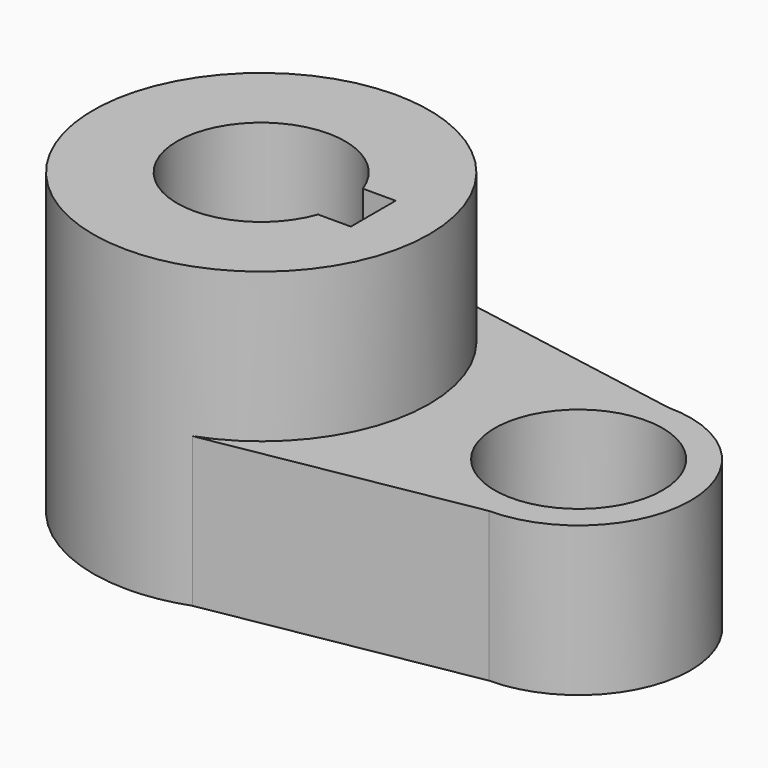
from build123d import *

# Parameters (mm, degrees)
F0_R     = 14.2875
F1_DEPTH = 25.4
F2_DEPTH = 50.8


with BuildPart() as f1:
    # F0 (on Top) → F1 (new body)
    with BuildSketch(Plane.XY):
        with BuildLine():
            Line((9.780704698, 26.8489932886), (0, 28.575))
            ThreePointArc((0, 28.575), (-28.575, 0), (0, -28.575))
            Line((0, -28.575), (9.780704698, -26.8489932886))
            ThreePointArc((9.780704698, -26.8489932886), (23.4095521288, -16.3866864902), (28.575, 0))
            ThreePointArc((28.575, 0), (23.4095521288, 16.3866864902), (9.780704698, 26.8489932886))
        make_face()
        with BuildLine():
            ThreePointArc((-13.4703841816, 4.7625), (0, 14.2875), (13.4703841816, 4.7625))
            Line((13.4703841816, 4.7625), (19.05, 4.7625))
            Line((19.05, 4.7625), (19.05, -4.7625))
            Line((19.05, -4.7625), (13.4703841816, -4.7625))
            ThreePointArc((13.4703841816, -4.7625), (0, -14.2875), (-13.4703841816, -4.7625))
            Line((-13.4703841816, -4.7625), (-19.05, -4.7625))
            Line((-19.05, -4.7625), (-19.05, 4.7625))
            Line((-19.05, 4.7625), (-13.4703841816, 4.7625))
        make_face(mode=Mode.SUBTRACT)
        with BuildLine():
            ThreePointArc((9.780704698, 26.8489932886), (4.9659159165, 28.1401901932), (0, 28.575))
            Line((0, 28.575), (9.780704698, 26.8489932886))
        make_face()
        with BuildLine():
            Line((53.975, 19.05), (9.780704698, 26.8489932886))
            ThreePointArc((9.780704698, 26.8489932886), (23.4095521288, 16.3866864902), (28.575, 0))
            ThreePointArc((28.575, 0), (23.4095521288, -16.3866864902), (9.780704698, -26.8489932886))
            Line((9.780704698, -26.8489932886), (53.975, -19.05))
            ThreePointArc((53.975, -19.05), (34.925, 0), (53.975, 19.05))
        make_face()
        with BuildLine():
            ThreePointArc((73.025, 0), (67.4453841816, 13.4703841816), (53.975, 19.05))
            ThreePointArc((53.975, 19.05), (34.925, 0), (53.975, -19.05))
            ThreePointArc((53.975, -19.05), (67.4453841816, -13.4703841816), (73.025, 0))
        make_face()
        with Locations((53.975, 0)):
            Circle(F0_R, mode=Mode.SUBTRACT)
        with BuildLine():
            ThreePointArc((-13.4703841816, -4.7625), (-14.2875, 0), (-13.4703841816, 4.7625))
            Line((-13.4703841816, 4.7625), (-19.05, 4.7625))
            Line((-19.05, 4.7625), (-19.05, -4.7625))
            Line((-19.05, -4.7625), (-13.4703841816, -4.7625))
        make_face()
    extrude(amount=F1_DEPTH)

    # F0 (on Top) → F2 (join)
    with BuildSketch(Plane.XY):
        with BuildLine():
            ThreePointArc((9.780704698, 26.8489932886), (4.9659159165, 28.1401901932), (0, 28.575))
            Line((0, 28.575), (9.780704698, 26.8489932886))
        make_face()
        with BuildLine():
            Line((9.780704698, -26.8489932886), (0, -28.575))
            ThreePointArc((0, -28.575), (4.9659159165, -28.1401901932), (9.780704698, -26.8489932886))
        make_face()
        with BuildLine():
            Line((9.780704698, 26.8489932886), (0, 28.575))
            ThreePointArc((0, 28.575), (-28.575, 0), (0, -28.575))
            Line((0, -28.575), (9.780704698, -26.8489932886))
            ThreePointArc((9.780704698, -26.8489932886), (23.4095521288, -16.3866864902), (28.575, 0))
            ThreePointArc((28.575, 0), (23.4095521288, 16.3866864902), (9.780704698, 26.8489932886))
        make_face()
        with BuildLine():
            ThreePointArc((-13.4703841816, 4.7625), (0, 14.2875), (13.4703841816, 4.7625))
            Line((13.4703841816, 4.7625), (19.05, 4.7625))
            Line((19.05, 4.7625), (19.05, -4.7625))
            Line((19.05, -4.7625), (13.4703841816, -4.7625))
            ThreePointArc((13.4703841816, -4.7625), (0, -14.2875), (-13.4703841816, -4.7625))
            Line((-13.4703841816, -4.7625), (-19.05, -4.7625))
            Line((-19.05, -4.7625), (-19.05, 4.7625))
            Line((-19.05, 4.7625), (-13.4703841816, 4.7625))
        make_face(mode=Mode.SUBTRACT)
        with BuildLine():
            ThreePointArc((-13.4703841816, -4.7625), (-14.2875, 0), (-13.4703841816, 4.7625))
            Line((-13.4703841816, 4.7625), (-19.05, 4.7625))
            Line((-19.05, 4.7625), (-19.05, -4.7625))
            Line((-19.05, -4.7625), (-13.4703841816, -4.7625))
        make_face()
    extrude(amount=F2_DEPTH)


solid = f1.part
